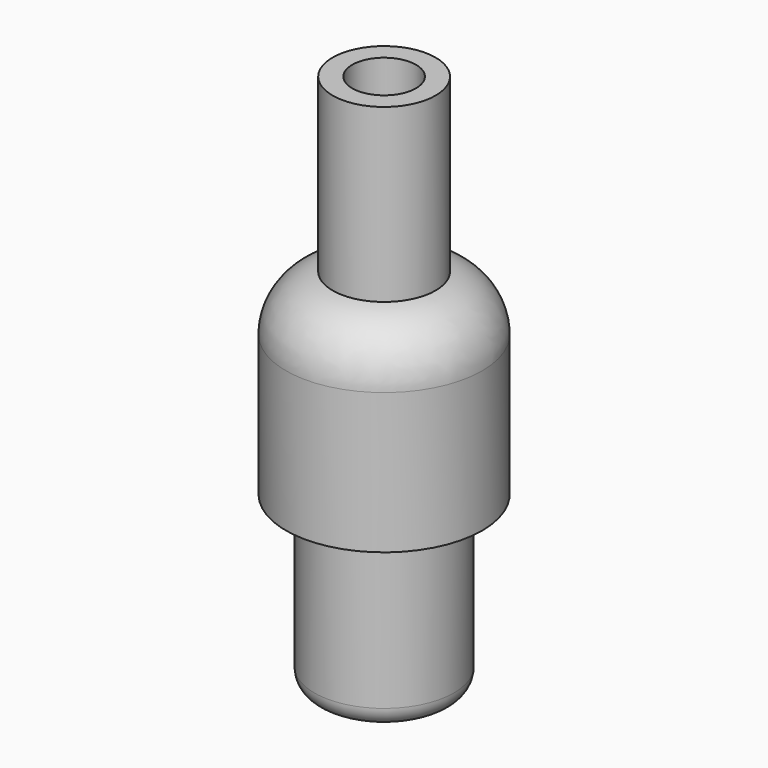
from build123d import *

# Parameters (mm, degrees)
F0_R     = 2.1
F0_R_2   = 1.3
F1_DEPTH = 15
F0_R_3   = 2.85
F2_DEPTH = 7
F0_R_4   = 4
F3_DEPTH = 8
F5_R     = 0.8


# Not quite as in the source:
# - a fillet or chamfer that OpenCascade refuses, or shapes differently, is made with other operations: its cross-section is extruded or revolved along the edge and cut away or added


with BuildPart() as f1:
    # F0 (on Top) → F1 (new body)
    with BuildSketch(Plane.XY):
        Circle(F0_R)
        Circle(F0_R_2, mode=Mode.SUBTRACT)
    extrude(amount=F1_DEPTH)

    # F0 (on Top) → F2 (join)
    with BuildSketch(Plane.XY):
        Circle(F0_R_3)
        Circle(F0_R, mode=Mode.SUBTRACT)
        Circle(F0_R)
        Circle(F0_R_2, mode=Mode.SUBTRACT)
    extrude(amount=-F2_DEPTH)

    # F0 (on Top) → F3 (join)
    with BuildSketch(Plane.XY):
        Circle(F0_R_4)
        Circle(F0_R_3, mode=Mode.SUBTRACT)
        Circle(F0_R_3)
        Circle(F0_R, mode=Mode.SUBTRACT)
    extrude(amount=F3_DEPTH)

    # F4: fillet of radius 2.3 on 1 edges, made by hand

    # F4_s1 → F4_t2 (revolve, cut)
    with BuildSketch(Plane.XZ):
        with BuildLine():
            ThreePointArc((2.1, 8), (3.4621010187, 7.2132242193), (4, 5.7350496694))
            Line((4, 5.7350496694), (4, 8))
            Line((4, 8), (2.1, 8))
        make_face()
    revolve(axis=Axis((0, 0, 8), (0, 0, 1)), mode=Mode.SUBTRACT)

    # F5
    f5_edges = [f1.edges().sort_by_distance(p)[0] for p in [
        (-2.85, 0, -7),
    ]]
    fillet(f5_edges, radius=F5_R)


solid = f1.part
